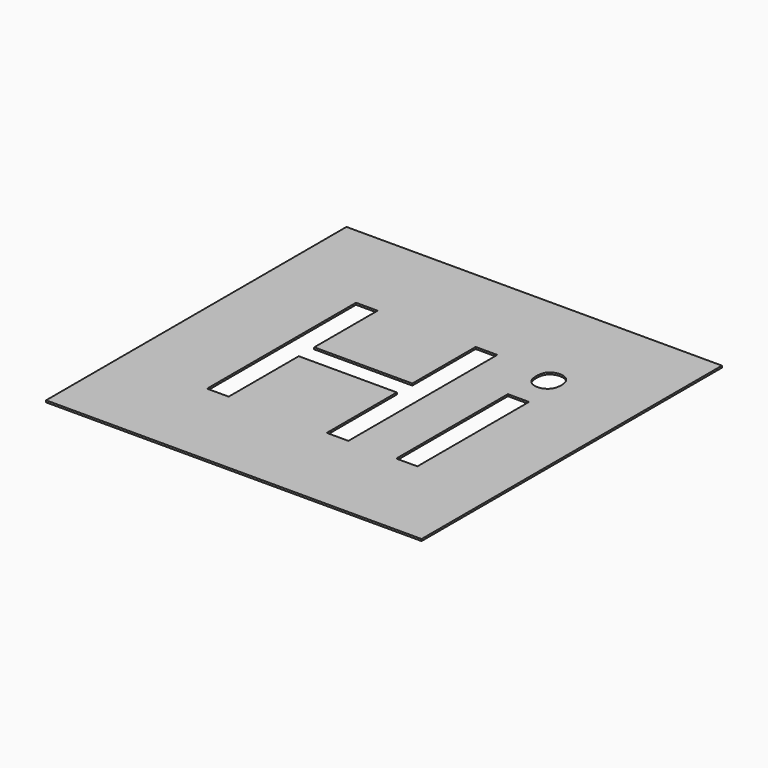
from build123d import *

# Parameters (mm, degrees)
F0_W         = 20
F0_H         = 20
F1_DEPTH     = 0.1
F2_TEXT_SIZE = 13.8888888889
F3_DEPTH     = 0.101


# Not quite as in the source:
# - Text() gives the source's letters only with a copy of the font that has no kerning and outlines rounded to 1/6400 em; it was checked with that copy


with BuildPart() as f1:
    # F0 (on Top) → F1 (new body)
    with BuildSketch(Plane.XY):
        with Locations((10, 10)):
            Rectangle(F0_W, F0_H)
    extrude(amount=F1_DEPTH)

    # F2 (on face) → F3 (cut, through all)
    with BuildSketch(Plane.XY.offset(0.1)):
        with Locations((3.2118055556, 5)):
            Text('Hi', F2_TEXT_SIZE, font='Open Sans', text_align=(TextAlign.LEFT, TextAlign.BOTTOM))
    extrude(amount=-F3_DEPTH, mode=Mode.SUBTRACT)


solid = f1.part
